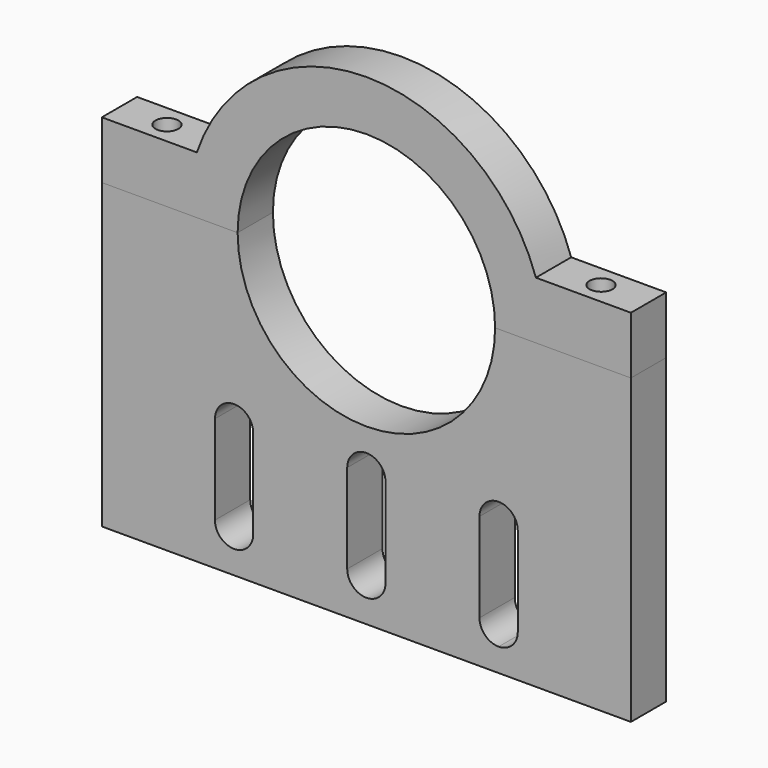
from build123d import *

# Parameters (mm, degrees)
F1_DEPTH         = 6.35
F2_DEPTH         = 6.35
F5_D             = 3.3
F5_DEPTH         = 19.05
F5_TIP           = 0.9914200214
F5_2_D           = 3.3
F5_2_DEPTH       = 19.05
F5_2_TIP         = 0.9914200214
F5_ON_F4_D       = 3.3
F5_ON_F4_DEPTH   = 19.05
F5_ON_F4_TIP     = 0.9914200214
F5_ON_F4_2_D     = 3.3
F5_ON_F4_2_DEPTH = 19.05
F5_ON_F4_2_TIP   = 0.9914200214


# Not quite as in the source:
# - a feature names something its author has since deleted; it is built from what else it names


with BuildPart() as f1:
    # F0 (on Front) → F1 (new body)
    with BuildSketch(Plane.XZ):
        with BuildLine():
            Line((-38.1, 0), (-38.1, -43.6063950042))
            Line((-38.1, -43.6063950042), (0, -43.6063950042))
            Line((0, -43.6063950042), (19.05, -43.6063950042))
            Line((19.05, -43.6063950042), (38.1, -43.6063950042))
            Line((38.1, -43.6063950042), (38.1, 0))
            Line((38.1, 0), (18.542, 0))
            ThreePointArc((18.542, 0), (0, -18.542), (-18.542, 0))
            Line((-18.542, 0), (-38.1, 0))
        make_face()
        with BuildLine():
            ThreePointArc((-21.8059, -24.6456172317), (-19.05, -21.8897172317), (-16.2941, -24.6456172317))
            Line((-16.2941, -24.6456172317), (-16.2941, -37.5027777724))
            ThreePointArc((-16.2941, -37.5027777724), (-19.05, -40.2586777724), (-21.8059, -37.5027777724))
            Line((-21.8059, -37.5027777724), (-21.8059, -24.6456172317))
        make_face(mode=Mode.SUBTRACT)
        with BuildLine():
            ThreePointArc((-2.7559, -24.6456172317), (0, -21.8897172317), (2.7559, -24.6456172317))
            Line((2.7559, -24.6456172317), (2.7559, -37.5027777724))
            ThreePointArc((2.7559, -37.5027777724), (0, -40.2586777724), (-2.7559, -37.5027777724))
            Line((-2.7559, -37.5027777724), (-2.7559, -24.6456172317))
        make_face(mode=Mode.SUBTRACT)
        with BuildLine():
            ThreePointArc((21.8059, -37.5027777724), (20.9987155783, -39.4514933507), (19.05, -40.2586777724))
            ThreePointArc((19.05, -40.2586777724), (17.1012844217, -39.4514933507), (16.2941, -37.5027777724))
            Line((16.2941, -37.5027777724), (16.2941, -24.6456172317))
            ThreePointArc((16.2941, -24.6456172317), (19.05, -21.8897172317), (21.8059, -24.6456172317))
            Line((21.8059, -24.6456172317), (21.8059, -37.5027777724))
        make_face(mode=Mode.SUBTRACT)
    extrude(amount=-F1_DEPTH)

    # F5
    with Locations(Plane.XY.offset(8.2744888681)):
        with Locations((-31.260012702, 3.175)):
            Hole(F5_D / 2, depth=F5_DEPTH)
            with Locations((0, 0, -(F5_DEPTH + F5_TIP / 2))):  # 118° drill point
                Cone(0, F5_D / 2, F5_TIP, mode=Mode.SUBTRACT)

    # F5 on F4
    with Locations(Plane.XY.offset(8.2744888681)):
        with Locations((31.260012702, 3.175)):
            Hole(F5_ON_F4_D / 2, depth=F5_ON_F4_DEPTH)
            with Locations((0, 0, -(F5_ON_F4_DEPTH + F5_ON_F4_TIP / 2))):  # 118° drill point
                Cone(0, F5_ON_F4_D / 2, F5_ON_F4_TIP, mode=Mode.SUBTRACT)


with BuildPart() as f2:
    # F0 (on Front) → F2 (new body)
    with BuildSketch(Plane.XZ):
        with BuildLine():
            Line((-38.1, 8.2744888681), (-38.1, 0))
            Line((-38.1, 0), (-18.542, 0))
            ThreePointArc((-18.542, 0), (0, 18.542), (18.542, 0))
            Line((18.542, 0), (38.1, 0))
            Line((38.1, 0), (38.1, 8.2744888681))
            Line((38.1, 8.2744888681), (24.4200254041, 8.2744888681))
            ThreePointArc((24.4200254041, 8.2744888681), (0, 25.7838090042), (-24.4200254041, 8.2744888681))
            Line((-24.4200254041, 8.2744888681), (-38.1, 8.2744888681))
        make_face()
    extrude(amount=-F2_DEPTH)

    # F5#2
    with Locations(Plane.XY.offset(8.2744888681)):
        with Locations((-31.260012702, 3.175)):
            Hole(F5_2_D / 2, depth=F5_2_DEPTH)
            with Locations((0, 0, -(F5_2_DEPTH + F5_2_TIP / 2))):  # 118° drill point
                Cone(0, F5_2_D / 2, F5_2_TIP, mode=Mode.SUBTRACT)

    # F5 on F4#2
    with Locations(Plane.XY.offset(8.2744888681)):
        with Locations((31.260012702, 3.175)):
            Hole(F5_ON_F4_2_D / 2, depth=F5_ON_F4_2_DEPTH)
            with Locations((0, 0, -(F5_ON_F4_2_DEPTH + F5_ON_F4_2_TIP / 2))):  # 118° drill point
                Cone(0, F5_ON_F4_2_D / 2, F5_ON_F4_2_TIP, mode=Mode.SUBTRACT)


solid = Compound([f1.part, f2.part])
